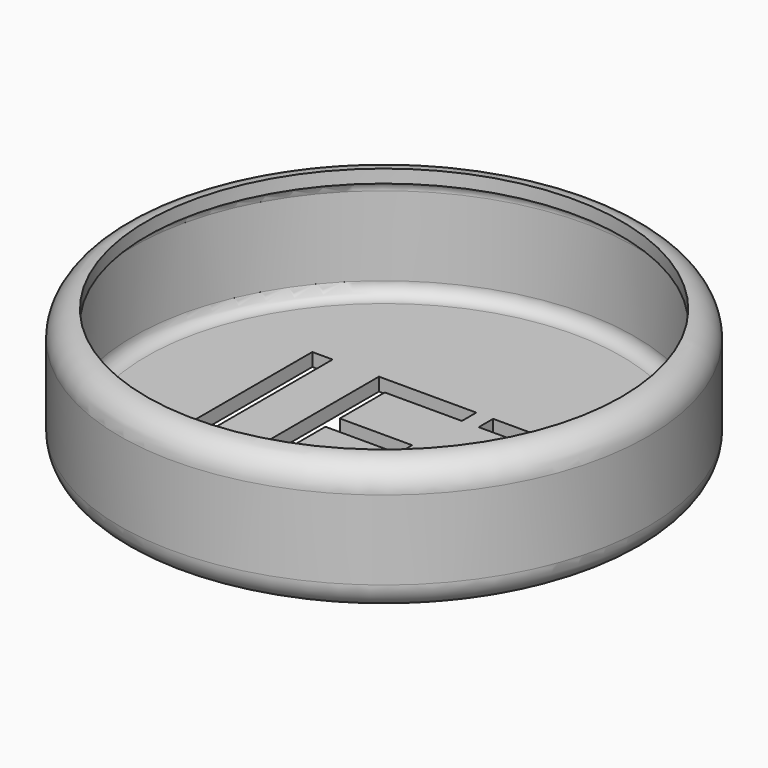
from build123d import *

# Parameters (mm, degrees)
F0_R         = 50
F1_DEPTH     = 25
F2_R         = 5
F3_T         = -2.5
F4_TEXT_SIZE = 46.357615894
F5_DEPTH     = 2.5


# Not quite as in the source:
# - a shell that OpenCascade refuses in one call is made with other operations: the cavity is built on its own and cut out
# - Text() gives the source's letters only with a copy of the font that has no kerning and outlines rounded to 1/6400 em; it was checked with that copy


with BuildPart() as f1:
    # F0 (on Top) → F1 (new body)
    with BuildSketch(Plane.XY):
        Circle(F0_R)
    extrude(amount=F1_DEPTH)

    # F2
    f2_edges = [f1.edges().sort_by_distance(p)[0] for p in [
        (-50, 0, 25),
        (-50, 0, 0),
    ]]
    fillet(f2_edges, radius=F2_R)

    # F3: a shell. OpenCascade refuses it in one call, so the cavity is built on its own and cut out:
    # the body offset inwards by the wall thickness, plus a prism from it out through each open face.
    f3_core = offset(f1.part, amount=F3_T, mode=Mode.PRIVATE)
    f3_exits = [f3_core.faces().sort_by_distance(p)[0] for p in [
        (0, 0, 22.5),
    ]]
    add(f3_core, mode=Mode.SUBTRACT)
    extrude(f3_exits, amount=-F3_T, mode=Mode.SUBTRACT)

    # F4 (on face) → F5 (cut, through all)
    with BuildSketch(Plane.XY.offset(2.5)):
        with Locations((-31, -16.7267727941)):
            Text('JET', F4_TEXT_SIZE, font='Open Sans', text_align=(TextAlign.LEFT, TextAlign.BOTTOM))
    extrude(amount=-F5_DEPTH, mode=Mode.SUBTRACT)


solid = f1.part
